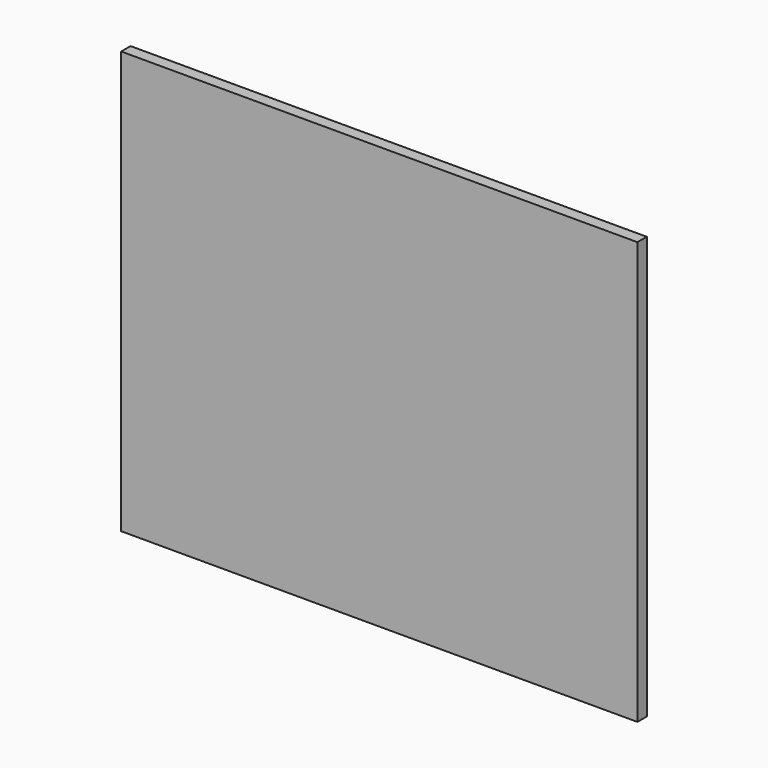
from build123d import *

# Parameters (mm, degrees)
F0_W     = 558.8
F0_H     = 457.2
F1_DEPTH = 12.7


# Not quite as in the source:
# - a length typed as a fraction of an inch, garbled in the dataset ("3 / 203.2 mm" for 3/8 in), is restored


with BuildPart() as f1:
    # F0 (on Front) → F1 (new body)
    with BuildSketch(Plane.XZ):
        Rectangle(F0_W, F0_H)
    extrude(amount=F1_DEPTH)


solid = f1.part
